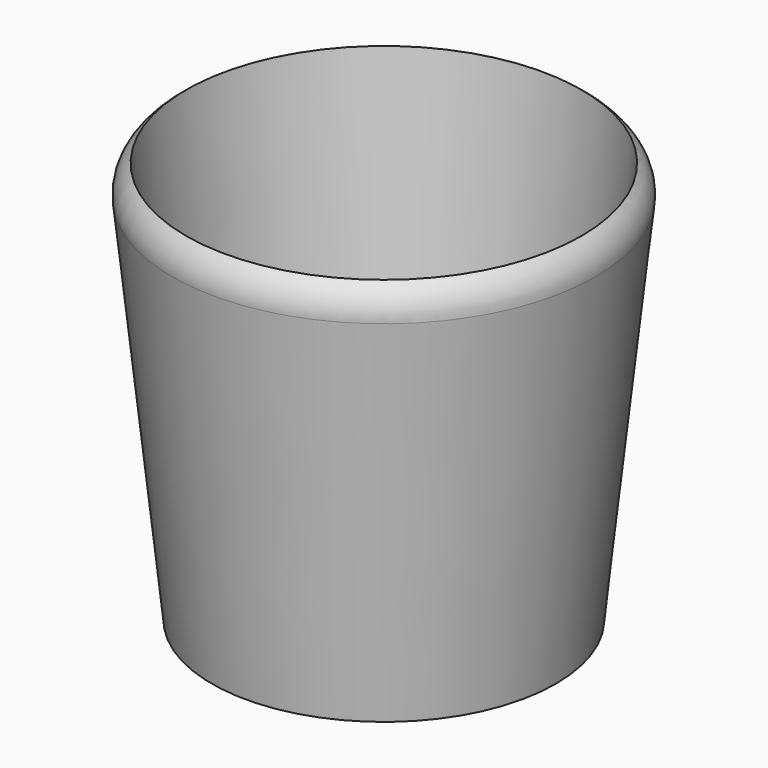
from build123d import *

# Parameters (mm, degrees)
F0_R = 25.4
F2_R = 31.75
F4_T = -2.54


# Not quite as in the source:
# - a fillet or chamfer that OpenCascade refuses, or shapes differently, is made with other operations: its cross-section is extruded or revolved along the edge and cut away or added


with BuildPart() as f3:
    # F0 (on Top) → F3 section 0
    with BuildSketch(Plane.XY):
        Circle(F0_R)
    # F2 (on offset) → F3 section 1
    with BuildSketch(Plane.XY.offset(59.436)):
        Circle(F2_R)
    loft()

    # F4
    f4_openings = [f3.faces().sort_by_distance(p)[0] for p in [
        (0, 0, 59.436),
    ]]
    offset(amount=F4_T, openings=f4_openings, kind=Kind.INTERSECTION)

    # F5: fillet of radius 5.08 on 1 edges, made by hand

    # F5_s1 → F5_t2 (revolve, cut)
    with BuildSketch(Plane.XZ):
        with BuildLine():
            ThreePointArc((31.2538092028, 54.7916541382), (30.8469014644, 57.3895821842), (29.195545003, 59.436))
            Line((29.195545003, 59.436), (31.75, 59.436))
            Line((31.75, 59.436), (31.2538092028, 54.7916541382))
        make_face()
    revolve(axis=Axis((0, 0, 59.436), (0, 0, 1)), mode=Mode.SUBTRACT)


solid = f3.part
